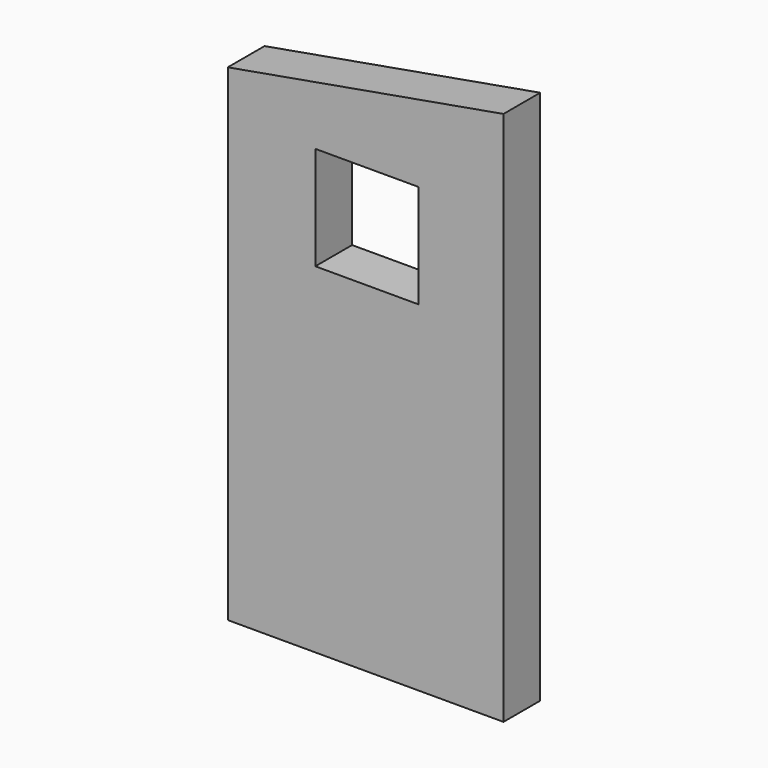
from build123d import *

# Parameters (mm, degrees)
F0_W        = 152.4
F0_H        = 304.8
F1_DEPTH    = 25.4
F2_T1_DEPTH = 1081.4461668656
F3_W        = 57.15
F3_H        = 57.15
F4_DEPTH    = 25.4


# Not quite as in the source:
# - a fillet or chamfer that OpenCascade refuses, or shapes differently, is made with other operations: its cross-section is extruded or revolved along the edge and cut away or added


with BuildPart() as f1:
    # F0 (on Front) → F1 (new body)
    with BuildSketch(Plane.XZ):
        with Locations((-29.3548897063, -4.3910965323)):
            Rectangle(F0_W, F0_H)
    extrude(amount=F1_DEPTH)

    # F2: chamfer of 203.2 x 35.82964248 on 1 edges, made by hand

    # F2_s2 → F2_t1 (cut)
    with BuildSketch(Plane.XZ.offset(-528.0230834328)):
        Polygon((97.6451102937, 148.0089034677), (-105.5548897063, 112.1792609877), (-105.5548897063, 148.0089034677), align=None)
    extrude(amount=F2_T1_DEPTH, mode=Mode.SUBTRACT)

    # F3 (on face) → F4 (cut, through all)
    with BuildSketch(Plane.XZ):
        with Locations((-28.575, 59.6764928477)):
            Rectangle(F3_W, F3_H)
    extrude(amount=F4_DEPTH, mode=Mode.SUBTRACT)


solid = f1.part
